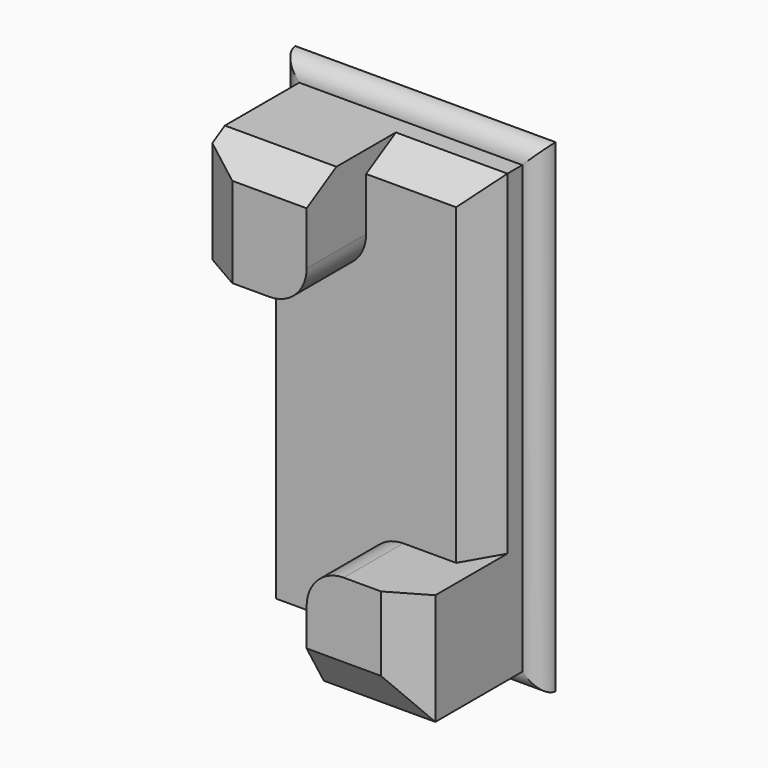
from build123d import *

# Parameters (mm, degrees)
F1_DEPTH    = 25.4
F2_DEPTH    = 50.8
F0_W        = 88.9
F0_H        = 165.1
F3_DEPTH    = 6.35
F4_C1_SIZE2 = 12.7
F4_C1_SIZE  = 7.3323484187
F4_C2_SIZE2 = 7.3323484187
F4_C2_SIZE  = 12.7
F4_C3_SIZE2 = 12.7
F4_C3_SIZE  = 7.3323484187
F4_C4_SIZE2 = 12.7
F4_C4_SIZE  = 7.3323484187
F5_C1_SIZE2 = 7.3323484187
F5_C1_SIZE  = 12.7
F5_C2_SIZE2 = 7.3323484187
F5_C2_SIZE  = 12.7
F5_C3_SIZE2 = 7.3323484187
F5_C3_SIZE  = 12.7
F5_C4_SIZE2 = 7.3323484187
F5_C4_SIZE  = 12.7
F6_R        = 6.34999


# Not quite as in the source:
# - a fillet or chamfer is up to 0.001 mm smaller than in the source, because OpenCascade refuses the exact size


with BuildPart() as f1:
    # F0 (on Front) → F1 (new body)
    with BuildSketch(Plane.XZ):
        with BuildLine():
            Line((38.1, 76.2), (0, 76.2))
            Line((0, 76.2), (0, 50.8))
            ThreePointArc((0, 50.8), (-3.7197438789, 41.8197438789), (-12.7, 38.1))
            Line((-12.7, 38.1), (-38.1, 38.1))
            Line((-38.1, 38.1), (-38.1, -76.2))
            Line((-38.1, -76.2), (0, -76.2))
            Line((0, -76.2), (0, -50.8))
            ThreePointArc((0, -50.8), (3.7197438789, -41.8197438789), (12.7, -38.1))
            Line((12.7, -38.1), (38.1, -38.1))
            Line((38.1, -38.1), (38.1, 76.2))
        make_face()
    extrude(amount=F1_DEPTH)

    # F0 (on Front) → F2 (join)
    with BuildSketch(Plane.XZ):
        with BuildLine():
            Line((38.1, -76.2), (38.1, -38.1))
            Line((38.1, -38.1), (12.7, -38.1))
            ThreePointArc((12.7, -38.1), (3.7197438789, -41.8197438789), (0, -50.8))
            Line((0, -50.8), (0, -76.2))
            Line((0, -76.2), (38.1, -76.2))
        make_face()
        with BuildLine():
            Line((0, 76.2), (-38.1, 76.2))
            Line((-38.1, 76.2), (-38.1, 38.1))
            Line((-38.1, 38.1), (-12.7, 38.1))
            ThreePointArc((-12.7, 38.1), (-3.7197438789, 41.8197438789), (0, 50.8))
            Line((0, 50.8), (0, 76.2))
        make_face()
    extrude(amount=F2_DEPTH)

    # F0 (on Front) → F3 (join)
    with BuildSketch(Plane.XZ):
        Rectangle(F0_W, F0_H)
        Polygon((-38.1, 38.1), (-38.1, 76.2), (0, 76.2), (38.1, 76.2), (38.1, -38.1), (38.1, -76.2), (0, -76.2), (-38.1, -76.2), align=None, mode=Mode.SUBTRACT)
    extrude(amount=F3_DEPTH)

    # F4: chamfer of 12.7 x 7.3323484187 on 4 edges, made by hand

    # F4_c1
    f4_c1_edges = [f1.edges().sort_by_distance(p)[0] for p in [
        (38.1, -50.8, -57.15),
    ]]
    f4_c1_side = f1.faces().sort_by_distance((38.1, -50.6533530316, -57.15))[0]
    chamfer(f4_c1_edges, length=F4_C1_SIZE, length2=F4_C1_SIZE2, reference=f4_c1_side)

    # F4_c2
    f4_c2_edges = [f1.edges().sort_by_distance(p)[0] for p in [
        (-19.05, -50.8, 76.2),
    ]]
    f4_c2_side = f1.faces().sort_by_distance((-19.05, -50.6533530316, 76.2))[0]
    chamfer(f4_c2_edges, length=F4_C2_SIZE, length2=F4_C2_SIZE2, reference=f4_c2_side)

    # F4_c3
    f4_c3_edges = [f1.edges().sort_by_distance(p)[0] for p in [
        (12.7, -50.8, -76.2),
    ]]
    f4_c3_side = f1.faces().sort_by_distance((12.7, -50.6533530316, -76.2))[0]
    chamfer(f4_c3_edges, length=F4_C3_SIZE, length2=F4_C3_SIZE2, reference=f4_c3_side)

    # F4_c4
    f4_c4_edges = [f1.edges().sort_by_distance(p)[0] for p in [
        (-38.1, -50.8, 53.4838257906),
    ]]
    f4_c4_side = f1.faces().sort_by_distance((-38.1, -50.6533530316, 53.4838257906))[0]
    chamfer(f4_c4_edges, length=F4_C4_SIZE, length2=F4_C4_SIZE2, reference=f4_c4_side)

    # F5: chamfer of 12.7 x 7.3323484187 on 4 edges, made by hand

    # F5_c1
    f5_c1_edges = [f1.edges().sort_by_distance(p)[0] for p in [
        (-38.1, -25.4, -19.05),
    ]]
    f5_c1_side = f1.faces().sort_by_distance((-38.1, -25.2533530316, -19.05))[0]
    chamfer(f5_c1_edges, length=F5_C1_SIZE, length2=F5_C1_SIZE2, reference=f5_c1_side)

    # F5_c2
    f5_c2_edges = [f1.edges().sort_by_distance(p)[0] for p in [
        (19.05, -25.4, 76.2),
    ]]
    f5_c2_side = f1.faces().sort_by_distance((19.05, -25.2533530316, 76.2))[0]
    chamfer(f5_c2_edges, length=F5_C2_SIZE, length2=F5_C2_SIZE2, reference=f5_c2_side)

    # F5_c3
    f5_c3_edges = [f1.edges().sort_by_distance(p)[0] for p in [
        (38.1, -25.4, 15.3838257906),
    ]]
    f5_c3_side = f1.faces().sort_by_distance((38.1, -25.2533530316, 15.3838257906))[0]
    chamfer(f5_c3_edges, length=F5_C3_SIZE, length2=F5_C3_SIZE2, reference=f5_c3_side)

    # F5_c4
    f5_c4_edges = [f1.edges().sort_by_distance(p)[0] for p in [
        (-15.3838257906, -25.4, -76.2),
    ]]
    f5_c4_side = f1.faces().sort_by_distance((-15.3838257906, -25.2533530316, -76.2))[0]
    chamfer(f5_c4_edges, length=F5_C4_SIZE, length2=F5_C4_SIZE2, reference=f5_c4_side)

    # F6 (radius 6.35 in the source; OpenCascade refuses exactly that, so slightly less here)
    f6_edges = [f1.edges().sort_by_distance(p)[0] for p in [
        (0, -6.35, -82.55),
        (-44.45, -6.35, 0),
        (0, -6.35, 82.55),
        (44.45, -6.35, 0),
    ]]
    fillet(f6_edges, radius=F6_R)


solid = f1.part
